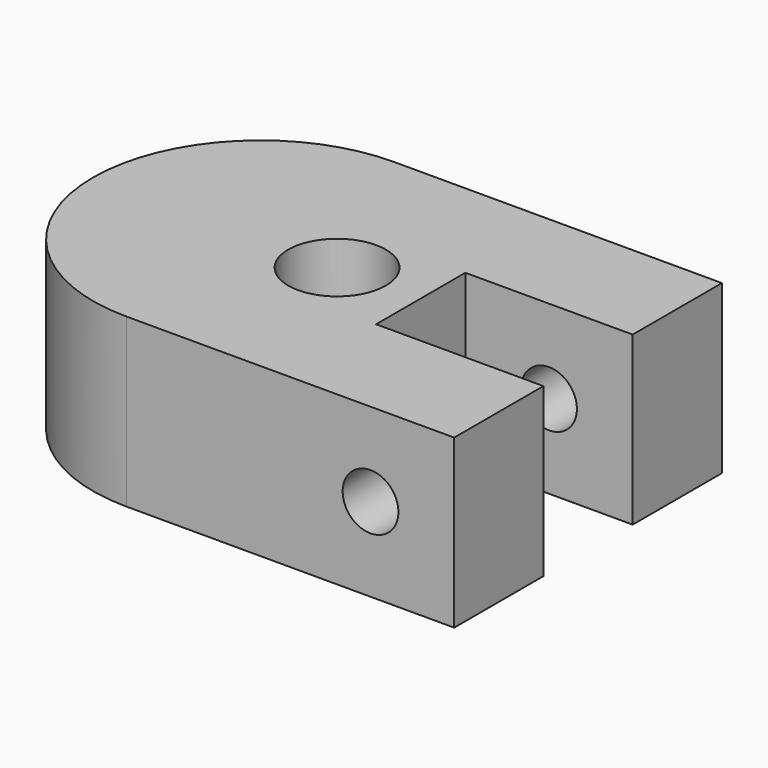
from build123d import *

# Parameters (mm, degrees)
F1_DEPTH = 76.2
F2_R     = 76.2
F3_R     = 76.19999
F5_R     = 12.7
F6_DEPTH = 152.4
F4_R     = 22.225
F7_DEPTH = 76.2


# Not quite as in the source:
# - a fillet or chamfer is up to 0.001 mm smaller than in the source, because OpenCascade refuses the exact size


with BuildPart() as f1:
    # F0 (on Top) → F1 (new body)
    with BuildSketch(Plane.XY):
        Polygon((0, 152.4), (0, 0), (225.425, 0), (225.425, 50.8), (149.225, 50.8), (149.225, 101.6), (225.425, 101.6), (225.425, 152.4), align=None)
    extrude(amount=F1_DEPTH)

    # F2
    f2_edges = [f1.edges().sort_by_distance(p)[0] for p in [
        (0, 152.4, 38.1),
    ]]
    fillet(f2_edges, radius=F2_R)

    # F3 (radius 76.2 in the source; OpenCascade refuses exactly that, so slightly less here)
    f3_edges = [f1.edges().sort_by_distance(p)[0] for p in [
        (0, 0, 38.1),
    ]]
    fillet(f3_edges, radius=F3_R)

    # F5 (on face) → F6 (cut)
    with BuildSketch(Plane(origin=(0, 152.4, 0), x_dir=(-1, 0, 0), z_dir=(0, 1, 0))):
        with Locations((-187.325, 38.1)):
            Circle(F5_R)
    extrude(amount=-F6_DEPTH, mode=Mode.SUBTRACT)

    # F4 (on face) → F7 (cut)
    with BuildSketch(Plane.XY.offset(76.2)):
        with Locations((111.125, 76.2)):
            Circle(F4_R)
    extrude(amount=-F7_DEPTH, mode=Mode.SUBTRACT)


solid = f1.part
